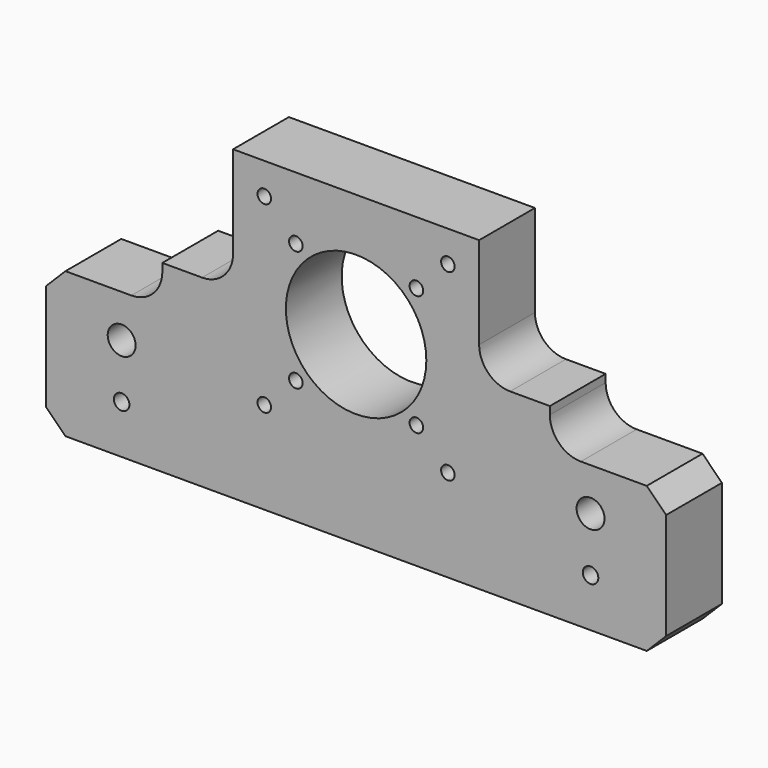
from build123d import *

# Parameters (mm, degrees)
F0_R           = 2
F0_W           = 63.5
F0_H           = 11.75
F0_R_2         = 1.75
F0_R_3         = 18.125
F1_DEPTH       = 18
F2_SIZE        = 5
F3_R           = 8
F4_D           = 7.2
F4_DEPTH       = 35
F4_CBORE_D     = 11
F4_CBORE_DEPTH = 6
F4_TIP         = 2.1630982285


with BuildPart() as f1:
    # F0 (on Front) → F1 (new body)
    with BuildSketch(Plane.XZ):
        Polygon((-80, -33.75), (80, -33.75), (80, 3.75), (50, 3.75), (50, 13.75), (31.75, 13.75), (31.75, -18), (-31.75, -18), (-31.75, 13.75), (-50, 13.75), (-50, 3.75), (-80, 3.75), align=None)
        with Locations((-60.5, -21.25)):
            Circle(F0_R, mode=Mode.SUBTRACT)
        with Locations((60.5, -21.25)):
            Circle(F0_R, mode=Mode.SUBTRACT)
        with Locations((0, 39.625)):
            Rectangle(F0_W, F0_H)
        with Locations((-23.6880771697, 37.4380771697)):
            Circle(F0_R_2, mode=Mode.SUBTRACT)
        with Locations((23.6880771697, 37.4380771697)):
            Circle(F0_R_2, mode=Mode.SUBTRACT)
        Polygon((31.75, 13.75), (31.75, 33.75), (-31.75, 33.75), (-31.75, 13.75), (-31.75, -18), (31.75, -18), align=None)
        with Locations((-23.6880771697, -9.9380771697)):
            Circle(F0_R_2, mode=Mode.SUBTRACT)
        with Locations((-15.5563491861, -1.8063491861)):
            Circle(F0_R_2, mode=Mode.SUBTRACT)
        with Locations((23.6880771697, -9.9380771697)):
            Circle(F0_R_2, mode=Mode.SUBTRACT)
        with Locations((15.5563491861, -1.8063491861)):
            Circle(F0_R_2, mode=Mode.SUBTRACT)
        with Locations((-15.5563491861, 29.3063491861)):
            Circle(F0_R_2, mode=Mode.SUBTRACT)
        with Locations((0, 13.75)):
            Circle(F0_R_3, mode=Mode.SUBTRACT)
        with Locations((15.5563491861, 29.3063491861)):
            Circle(F0_R_2, mode=Mode.SUBTRACT)
    extrude(amount=F1_DEPTH)

    # F2
    f2_edges = [f1.edges().sort_by_distance(p)[0] for p in [
        (-80, -9, -33.75),
        (80, -9, -33.75),
        (80, -9, 3.75),
        (-80, -9, 3.75),
    ]]
    chamfer(f2_edges, length=F2_SIZE)

    # F3
    f3_edges = [f1.edges().sort_by_distance(p)[0] for p in [
        (31.75, -9, 13.75),
        (-31.75, -9, 13.75),
        (50, -9, 3.75),
        (-50, -9, 3.75),
    ]]
    fillet(f3_edges, radius=F3_R)

    # F4
    with Locations(Plane(origin=(0, 0, 0), x_dir=(1, 0, 0), z_dir=(0, 1, 0))):
        with Locations((60.5, 7.25), (-60.5, 7.25)):
            CounterBoreHole(F4_D / 2, F4_CBORE_D / 2, F4_CBORE_DEPTH, depth=F4_DEPTH)
            with Locations((0, 0, -(F4_DEPTH + F4_TIP / 2))):  # 118° drill point
                Cone(0, F4_D / 2, F4_TIP, mode=Mode.SUBTRACT)


solid = f1.part
